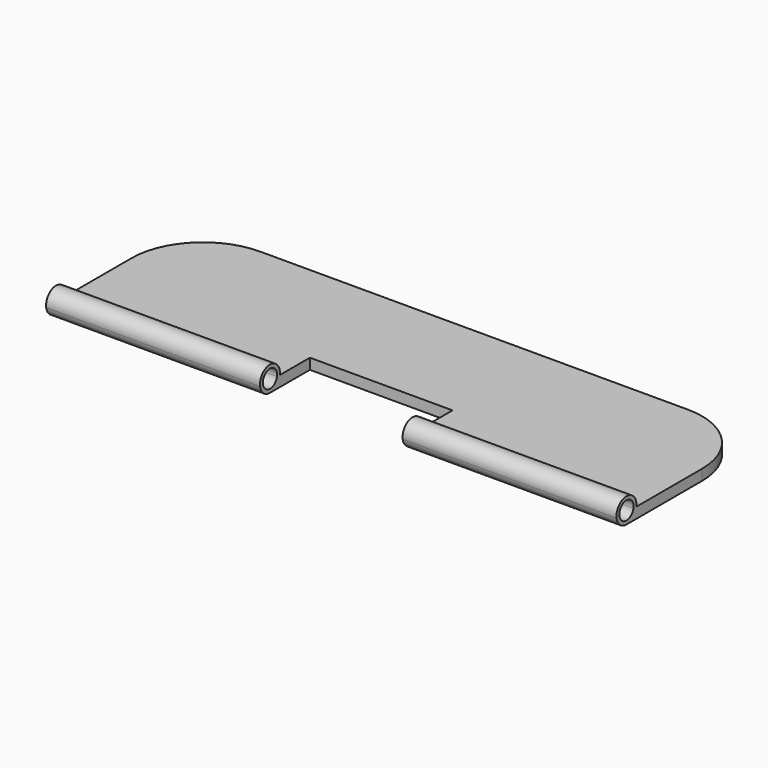
from build123d import *

# Parameters (mm, degrees)
F0_W      = 80
F0_H      = 25
F1_DEPTH  = 1.5
F2_R      = 10
F4_DEPTH  = 80
F3_R      = 1.75
F3_R_2    = 1.25
F5_DEPTH  = 80
F6_DEPTH  = 80
F7_W      = 20
F7_H      = 18.6819097605
F7_H_2    = 7
F8_DEPTH  = 25
F10_DEPTH = 0.5
F11_R     = 0.49999


# Not quite as in the source:
# - a fillet or chamfer is up to 0.001 mm smaller than in the source, because OpenCascade refuses the exact size


with BuildPart() as f1:
    # F0 (on Top) → F1 (new body)
    with BuildSketch(Plane.XY):
        Rectangle(F0_W, F0_H)
    extrude(amount=F1_DEPTH)

    # F2
    f2_edges = [f1.edges().sort_by_distance(p)[0] for p in [
        (-40, 12.5, 0.75),
        (40, 12.5, 0.75),
    ]]
    fillet(f2_edges, radius=F2_R)

    # F3 (on face) → F4 (cut)
    with BuildSketch(Plane(origin=(-40, 0, 0), x_dir=(0, -1, 0), z_dir=(-1, 0, 0))):
        with BuildLine():
            Line((12.5, 1.5), (12.4820508076, 1.5))
            ThreePointArc((12.4820508076, 1.5), (11.8956439237, 0.4271243445), (10.75, 0))
            Line((10.75, 0), (12.5, 0))
            Line((12.5, 0), (12.5, 1.5))
        make_face()
        with BuildLine():
            ThreePointArc((12.4820508076, 1.5), (12.495506934, 1.6246782406), (12.5, 1.75))
            ThreePointArc((12.5, 1.75), (10.6246782406, 3.495506934), (9.0179491924, 1.5))
            Line((9.0179491924, 1.5), (9.5252551286, 1.5))
            ThreePointArc((9.5252551286, 1.5), (10.6243637975, 2.9936701913), (12, 1.75))
            ThreePointArc((12, 1.75), (11.9936701913, 1.6243637975), (11.9747448714, 1.5))
            Line((11.9747448714, 1.5), (12.4820508076, 1.5))
        make_face()
    extrude(amount=-F4_DEPTH, mode=Mode.SUBTRACT)

    # F3 (on face) → F5 (join)
    with BuildSketch(Plane(origin=(-40, 0, 0), x_dir=(0, -1, 0), z_dir=(-1, 0, 0))):
        with Locations((10.75, 1.75)):
            Circle(F3_R)
        with Locations((10.75, 1.75)):
            Circle(F3_R_2, mode=Mode.SUBTRACT)
    extrude(amount=-F5_DEPTH)

    # F3 (on face) → F6 (cut)
    with BuildSketch(Plane(origin=(-40, 0, 0), x_dir=(0, -1, 0), z_dir=(-1, 0, 0))):
        with BuildLine():
            Line((11.9747448714, 1.5), (9.5252551286, 1.5))
            ThreePointArc((9.5252551286, 1.5), (10.75, 0.5), (11.9747448714, 1.5))
        make_face()
        with BuildLine():
            ThreePointArc((12, 1.75), (10.6243637975, 2.9936701913), (9.5252551286, 1.5))
            Line((9.5252551286, 1.5), (11.9747448714, 1.5))
            ThreePointArc((11.9747448714, 1.5), (11.9936701913, 1.6243637975), (12, 1.75))
        make_face()
    extrude(amount=-F6_DEPTH, mode=Mode.SUBTRACT)

    # F7 (on face) → F8 (cut)
    with BuildSketch(Plane(origin=(0, 0, 0), x_dir=(1, 0, 0), z_dir=(0, 0, -1))):
        with Locations((0, 20.0909548802)):
            Rectangle(F7_W, F7_H)
        with Locations((0, 7.25)):
            Rectangle(F7_W, F7_H_2)
    extrude(amount=-F8_DEPTH, mode=Mode.SUBTRACT)

    # F9 (on face) → F10 (join)
    with BuildSketch(Plane(origin=(0, 0, 0), x_dir=(1, 0, 0), z_dir=(0, 0, -1))):
        with BuildLine():
            Line((-36, 8.5), (-37, 8.5))
            Line((-37, 8.5), (-37, 0.5))
            ThreePointArc((-37, 0.5), (-34.0710678119, -6.5710678119), (-27, -9.5))
            Line((-27, -9.5), (-7, -9.5))
            Line((-7, -9.5), (-7, 0.5))
            Line((-7, 0.5), (-8, 0.5))
            Line((-8, 0.5), (-8, -8.5))
            Line((-8, -8.5), (-27, -8.5))
            ThreePointArc((-27, -8.5), (-33.3639610307, -5.8639610307), (-36, 0.5))
            Line((-36, 0.5), (-36, 8.5))
        make_face()
        with BuildLine():
            Line((8, 0.5), (7, 0.5))
            Line((7, 0.5), (7, -9.5))
            Line((7, -9.5), (27, -9.5))
            ThreePointArc((27, -9.5), (34.0710678119, -6.5710678119), (37, 0.5))
            Line((37, 0.5), (37, 8.5))
            Line((37, 8.5), (36, 8.5))
            Line((36, 8.5), (36, 0.5))
            ThreePointArc((36, 0.5), (33.3639610307, -5.8639610307), (27, -8.5))
            Line((27, -8.5), (8, -8.5))
            Line((8, -8.5), (8, 0.5))
        make_face()
    extrude(amount=F10_DEPTH)

    # F11 (radius 0.5 in the source; OpenCascade refuses exactly that, so slightly less here)
    f11_edges = [f1.edges().sort_by_distance(p)[0] for p in [
        (-36, -4.5, -0.5),
        (-36.5, -8.5, -0.5),
        (-37, -4.5, -0.5),
        (-34.071068, 6.571068, -0.5),
        (-17, 9.5, -0.5),
        (-7, 4.5, -0.5),
        (-7.5, -0.5, -0.5),
        (-8, 4, -0.5),
        (-17.5, 8.5, -0.5),
        (-33.363961, 5.863961, -0.5),
        (17.5, 8.5, -0.5),
        (8, 4, -0.5),
        (7.5, -0.5, -0.5),
        (7, 4.5, -0.5),
        (17, 9.5, -0.5),
        (34.071068, 6.571068, -0.5),
        (37, -4.5, -0.5),
        (36.5, -8.5, -0.5),
        (36, -4.5, -0.5),
        (33.363961, 5.863961, -0.5),
    ]]
    fillet(f11_edges, radius=F11_R)


solid = f1.part
